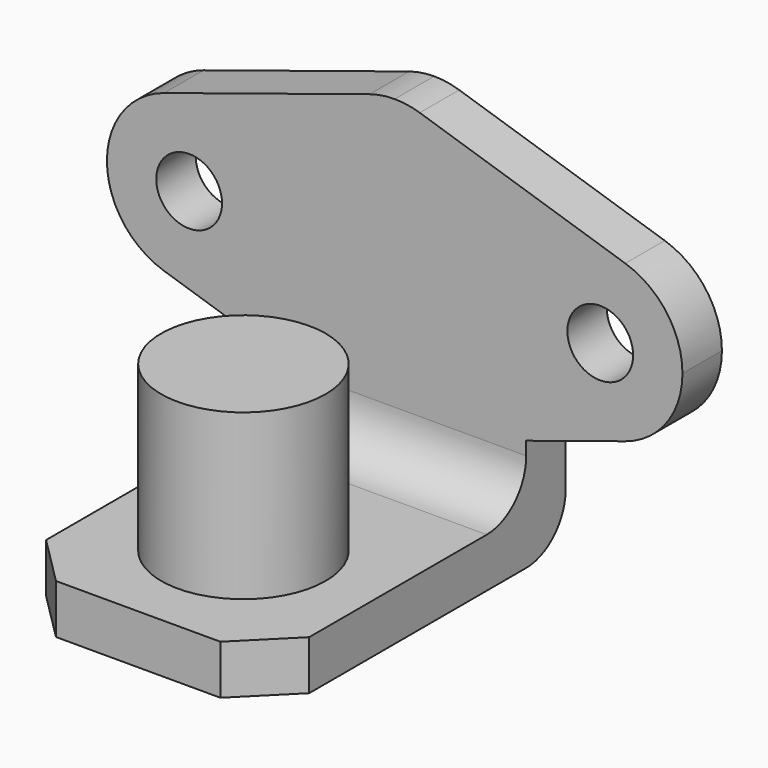
from build123d import *

# Parameters (mm, degrees)
F1_DEPTH = 70
F2_R     = 4
F3_DEPTH = 45.001
F4_R     = 8
F5_DEPTH = 45.001


with BuildPart() as f1:
    # F0 (on Right) → F1 (new body)
    with BuildSketch(Plane.YZ):
        with BuildLine():
            Line((0, 6), (0, 0))
            Line((0, 0), (39, 0))
            ThreePointArc((39, 0), (43.2426406871, 1.7573593129), (45, 6))
            Line((45, 6), (45, 45))
            Line((45, 45), (39, 45))
            Line((39, 45), (39, 12))
            ThreePointArc((39, 12), (37.2426406871, 7.7573593129), (33, 6))
            Line((33, 6), (0, 6))
        make_face()
    extrude(amount=F1_DEPTH)

    # F2 (on Front) → F3 (cut, through all)
    with BuildSketch(Plane.XZ):
        with Locations((10, 27)):
            Circle(F2_R)
        with Locations((60, 27)):
            Circle(F2_R)
        with BuildLine():
            ThreePointArc((63.047757271, 36.524241472), (68.0770530737, 32.8958641135), (70, 27))
            Line((70, 27), (70, 45))
            Line((70, 45), (35, 45))
            ThreePointArc((35, 45), (36.5423335048, 44.880344496), (38.047757271, 44.524241472))
            Line((38.047757271, 44.524241472), (63.047757271, 36.524241472))
        make_face()
        with BuildLine():
            Line((51, 13.620400082), (51, 0))
            Line((51, 0), (70, 0))
            Line((70, 0), (70, 27))
            ThreePointArc((70, 27), (68.0770699689, 21.1041590322), (63.0478118565, 17.4757759955))
            Line((63.0478118565, 17.4757759955), (51, 13.620400082))
        make_face()
        with BuildLine():
            Line((0, 0), (19, 0))
            Line((19, 0), (19, 13.620400082))
            Line((19, 13.620400082), (6.9521881435, 17.4757759955))
            ThreePointArc((6.9521881435, 17.4757759955), (1.922930031, 21.1041590323), (0, 27.0000000001))
            Line((0, 27.0000000001), (0, 0))
        make_face()
        with BuildLine():
            Line((0, 45), (0, 27.0000000001))
            ThreePointArc((0, 27.0000000001), (1.9229469263, 32.8958641136), (6.952242729, 36.524241472))
            Line((6.952242729, 36.524241472), (31.952242729, 44.524241472))
            ThreePointArc((31.952242729, 44.524241472), (33.4576664952, 44.880344496), (35, 45))
            Line((35, 45), (0, 45))
        make_face()
    extrude(amount=-F3_DEPTH, mode=Mode.SUBTRACT)

    # F4 (on Top) → F5 (cut, through all)
    with BuildSketch(Plane.XY):
        with Locations((35, 16)):
            Circle(F4_R)
        Polygon((19, 0), (25, 0), (19, 6), align=None)
        Polygon((45, 0), (51, 0), (51, 6), align=None)
    extrude(amount=F5_DEPTH, mode=Mode.SUBTRACT)

    # F7 (on offset) → F8 (revolve)
    with BuildSketch(Plane.XZ.offset(-16)):
        Polygon((35, 26), (35, 0), (43, 0), (43, 6), (45, 6), (45, 26), align=None)
    revolve(axis=Axis((35, 16, 13), (0, 0, 1)))


solid = f1.part
